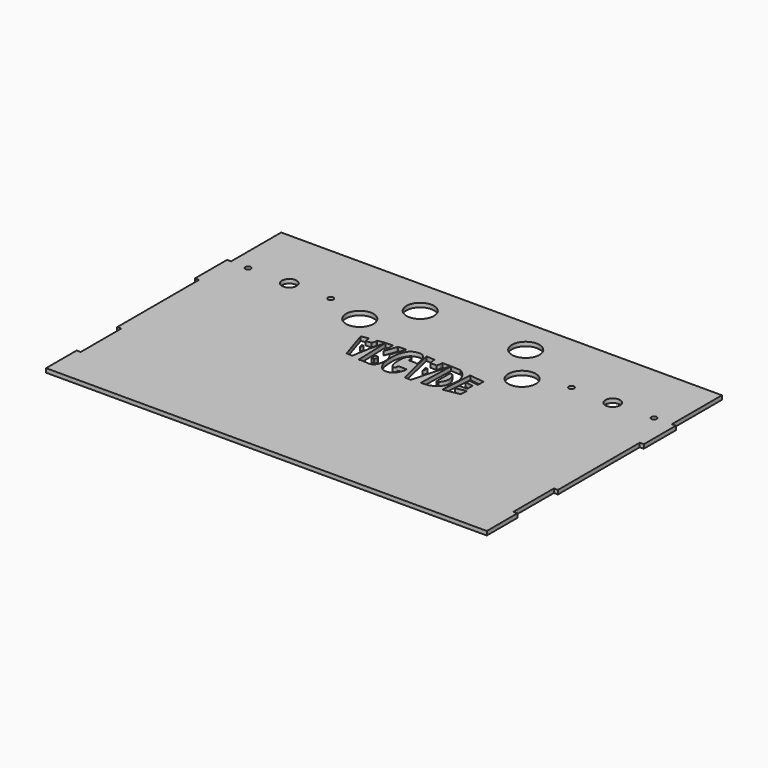
from build123d import *

# Parameters (mm, degrees)
F0_R     = 15.1
F0_R_2   = 3
F0_R_3   = 8.087272744
F1_DEPTH = 4.45


with BuildPart() as f1:
    # F0 (on Top) → F1 (new body)
    with BuildSketch(Plane.XY):
        Polygon((242.45, -33.63343), (238, -33.63343), (238, -28.2489694095), (238, 22.07074), (242.45, 22.07074), (242.45, 75.69707), (242.45, 134.5946788788), (246.9, 134.5946788788), (246.9, 178.6983170484), (242.45, 178.6983170484), (242.45, 237.5959259272), (242.45, 247.5959259272), (232.45, 247.5959259272), (-232.45, 247.5959259272), (-242.45, 247.5959259272), (-242.45, 237.5959259272), (-242.45, 178.6983170484), (-246.9, 178.6983170484), (-246.9, 134.5946788788), (-242.45, 134.5946788788), (-242.45, 75.69707), (-242.45, 22.07074), (-238, 22.07074), (-238, -33.63343), (-242.45, -33.63343), (-242.45, -75.69707), (-238, -75.69707), (238, -75.69707), (242.45, -75.69707), align=None)
        Polygon((-68.4135630727, 139.3414214253), (-60.2899454534, 140.9608349204), (-60.2899454534, 138.5317146778), (-59.6961602569, 135.2928876877), (-53.5423867404, 135.8326971531), (-52.3548163474, 139.611326158), (-52.3548163474, 141.8785080314), (-44.6356087923, 143.3311876865), (-44.6356087923, 140.1511281729), (-48.1983199716, 126.0622292757), (-51.5451095998, 106.4673140645), (-58.0227673054, 107.1690618992), (-62.3412020504, 120.5022409558), (-66.2278011441, 132.4859037995), (-67.6852688193, 137.6140490174), align=None, mode=Mode.SUBTRACT)
        with BuildLine():
            add(Edge.make_bspline(
                [(-27.7944092972, 128.5793082409), (-27.0867796861, 127.9867854546), (-26.5207327972, 126.9809206754), (-26.0123479414, 126.0622292782)],
                knots=[0.9431341245, 0.9431341245, 0.9431341245, 0.9431341245, 1, 1, 1, 1], degree=3))
            add(Edge.make_bspline(
                [(-26.0123479414, 126.0622292782), (-24.9726421233, 124.183399136), (-24.1741076418, 122.6691714867), (-23.7052644837, 120.7018569136)],
                knots=[0, 0, 0, 0, 0.1162972911, 0.1162972911, 0.1162972911, 0.1162972911], degree=3))
            add(Edge.make_bspline(
                [(-23.7052644837, 120.7018569136), (-23.1375532635, 118.3196816861), (-22.9666166078, 112.1430032153), (-27.438275439, 101.9479490434), (-39.3040642123, 106.008225837), (-42.5458674044, 104.0137255763), (-42.6923110384, 104.9558669353)],
                knots=[0.1162972911, 0.1162972911, 0.1162972911, 0.1162972911, 0.2571189623, 0.4018084692, 0.5633484367, 0.6431910445, 0.6431910445, 0.6431910445, 0.6431910445], degree=3))
            add(Edge.make_bspline(
                [(-42.6923110384, 104.9558669353), (-42.7094926771, 105.0664045668), (-42.7139295815, 105.1989924947), (-42.7063165735, 105.351943218)],
                knots=[0.6431910445, 0.6431910445, 0.6431910445, 0.6431910445, 0.6525586544, 0.6525586544, 0.6525586544, 0.6525586544], degree=3))
            Line((-42.7063165735, 105.351943218), (-44.0418235958, 143.1200578809))
            Line((-44.0418235958, 143.1200578809), (-36.0956337116, 143.401040728))
            Line((-36.0956337116, 143.401040728), (-36.0956337116, 130.2187219407))
            Line((-36.0956337116, 130.2187219407), (-31.5723344689, 142.5802558806))
            Line((-31.5723344689, 142.5802558806), (-31.2609091575, 144.1373843915))
            Line((-31.2609091575, 144.1373843915), (-22.0717723521, 144.793450565))
            Line((-22.0717723521, 144.793450565), (-27.7944092972, 128.5793082409))
        make_face(mode=Mode.SUBTRACT)
        with BuildLine():
            add(Edge.make_bspline(
                [(-8.3987614374, 115.9079596425), (-8.8505736963, 115.5068793363), (-8.2203283958, 114.0237563809), (-9.2346055247, 112.1843642837), (-11.1231552667, 111.810401025), (-13.0410600618, 113.3805151721), (-14.7964680369, 119.6526358134), (-14.9734613535, 125.835496877), (-14.3598206307, 132.1126885852), (-12.600885128, 135.7797795043), (-9.2769967864, 136.3883881539), (-8.7677567263, 133.3151455163), (-7.9106360899, 129.8026476212), (-6.8851230427, 130.3783952995), (-0.1435064114, 130.5317951707), (2.2047108084, 129.0160512993), (-0.9344140221, 140.8064141996), (-1.4129937988, 140.7859317655), (-4.7779902553, 147.2185915739), (-13.5960178433, 146.1939684974), (-18.7796230071, 143.3240652812), (-22.8561119513, 135.0899237079), (-23.625439333, 124.2814713806), (-22.4839389086, 112.4683388285), (-18.4573892555, 105.9850491154), (-14.5083812426, 102.0032027615), (-9.6389238746, 101.8342302081), (-4.2200323299, 103.0380617438), (-0.266790425, 109.186277671), (0.8380024016, 114.4887293174), (1.2785639857, 116.2657429546), (-1.4562686379, 115.9183349605), (-7.5129956046, 116.6942668408), (-8.3987614374, 115.9079596425)],
                knots=[0, 0, 0, 0, 0.020494547, 0.0414693591, 0.0607350939, 0.0828404788, 0.1209521426, 0.159932456, 0.1980232824, 0.2276772762, 0.2510011815, 0.2764947931, 0.3037065377, 0.3173900946, 0.3574312462, 0.3741991924, 0.4232910827, 0.4368372532, 0.4735096835, 0.516799885, 0.5533151147, 0.5976483724, 0.648419728, 0.7005614172, 0.7421530316, 0.776720808, 0.8090959926, 0.8438514827, 0.8845213381, 0.9201032118, 0.9362852602, 0.9598209895, 1, 1, 1, 1], degree=3))
        make_face(mode=Mode.SUBTRACT)
        with Locations((-89.2705285023, 164.2249039248)):
            Circle(F0_R, mode=Mode.SUBTRACT)
        with Locations((-223.3317792416, 178.1980395317)):
            Circle(F0_R_2, mode=Mode.SUBTRACT)
        with Locations((-177.8817792416, 178.1980395317)):
            Circle(F0_R_3, mode=Mode.SUBTRACT)
        with BuildLine():
            ThreePointArc((-135.4317792416, 178.1980395317), (-132.4317792416, 181.1980395317), (-129.4317792416, 178.1980395317))
            ThreePointArc((-129.4317792416, 178.1980395317), (-132.4317792416, 175.1980395317), (-135.4317792416, 178.1980395317))
        make_face(mode=Mode.SUBTRACT)
        with Locations((-58.0227673054, 208.2941681147)):
            Circle(F0_R, mode=Mode.SUBTRACT)
        Polygon((26.5557151985, 144.4220393921), (26.6185459447, 143.7345147158), (15.7999546033, 103.1001955295), (8.8810902786, 103.1001955295), (-0.9311196221, 144.9999362255), (-0.9311196221, 145.5496400619), (-0.532409514, 145.5496400619), (8.3791912299, 145.024992528), (8.3791912299, 142.775356772), (9.6371668157, 137.8542408372), (16.4302346062, 137.8542408372), (17.4366161924, 142.142631116), (17.4366161924, 144.4220393921), align=None, mode=Mode.SUBTRACT)
        with BuildLine():
            Line((25.9928592246, 103.9922162915), (27.0943791371, 144.4220393921))
            Line((27.0943791371, 144.4220393921), (38.1948985856, 143.7345147158))
            ThreePointArc((38.1948985856, 143.7345147158), (48.7228479864, 122.9251507383), (34.2359357279, 104.649573567))
            Line((34.2359357279, 104.649573567), (25.9928592246, 103.9922162915))
        make_face(mode=Mode.SUBTRACT)
        Polygon((56.2161091041, 133.1707835222), (55.5815506879, 128.7712032755), (64.17520246, 127.5317272908), (64.17520246, 120.3407719756), (55.311195622, 120.3407719756), (55.311195622, 114.7517710949), (66.5771887403, 116.9659271861), (66.0115630132, 108.9449003363), (48.2489814485, 105.7801532266), (50.5962303516, 141.4800577086), (66.7552874189, 139.1906589294), (66.7552874189, 131.6507011677), align=None, mode=Mode.SUBTRACT)
        with Locations((89.2705285023, 164.2249039248)):
            Circle(F0_R, mode=Mode.SUBTRACT)
        with Locations((58.0227673054, 208.2941681147)):
            Circle(F0_R, mode=Mode.SUBTRACT)
        with Locations((132.4317792416, 178.1980395317)):
            Circle(F0_R_2, mode=Mode.SUBTRACT)
        with Locations((177.8817792416, 178.1980395317)):
            Circle(F0_R_3, mode=Mode.SUBTRACT)
        with Locations((223.3317792416, 178.1980395317)):
            Circle(F0_R_2, mode=Mode.SUBTRACT)
        with BuildLine():
            Line((-27.7944092972, 128.5793082409), (-27.9016624439, 128.2754242445))
            Line((-27.9016624439, 128.2754242445), (-26.0123479414, 126.0622292782))
            add(Edge.make_bspline(
                [(-27.7944092972, 128.5793082409), (-27.0867796861, 127.9867854546), (-26.5207327972, 126.9809206754), (-26.0123479414, 126.0622292782)],
                knots=[0.9431341245, 0.9431341245, 0.9431341245, 0.9431341245, 1, 1, 1, 1], degree=3))
        make_face()
    extrude(amount=F1_DEPTH)


with BuildPart() as f1b:
    # F0 (on Top) → F1, piece 2 (new body)
    with BuildSketch(Plane.XY):
        Polygon((-33.2049726743, 119.1954817825), (-36.1722478731, 119.1954817825), (-35.9707883793, 113.4982109094), (-33.2049726743, 113.841682675), (-32.5294469364, 114.7517710949), (-32.2305089116, 115.8745737529), (-32.1074257839, 117.619991305), align=None)
    extrude(amount=F1_DEPTH)


with BuildPart() as f1c:
    # F0 (on Top) → F1, piece 3 (new body)
    with BuildSketch(Plane.XY):
        Polygon((12.8990933996, 122.5531250263), (14.2085683298, 128.3120363975), (11.5896194008, 128.3120363975), align=None)
    extrude(amount=F1_DEPTH)


with BuildPart() as f1d:
    # F0 (on Top) → F1, piece 4 (new body)
    with BuildSketch(Plane.XY):
        with BuildLine():
            Line((34.6707255345, 114.7517710949), (36.8092843097, 114.7517710949))
            ThreePointArc((36.8092843097, 114.7517710949), (40.9329586351, 123.8554957905), (37.3124741715, 133.1707835222))
            Line((37.3124741715, 133.1707835222), (34.6707255345, 133.4519907857))
            Line((34.6707255345, 133.4519907857), (34.6707255345, 114.7517710949))
        make_face()
    extrude(amount=F1_DEPTH)


with BuildPart() as f1e:
    # F0 (on Top) → F1, piece 5 (new body)
    with BuildSketch(Plane.XY):
        Polygon((-57.658851077, 127.3644715572), (-56.3293322224, 123.1370642806), (-55.5041096408, 127.3644715572), align=None)
    extrude(amount=F1_DEPTH)


solid = Compound([f1.part, f1b.part, f1c.part, f1d.part, f1e.part])
